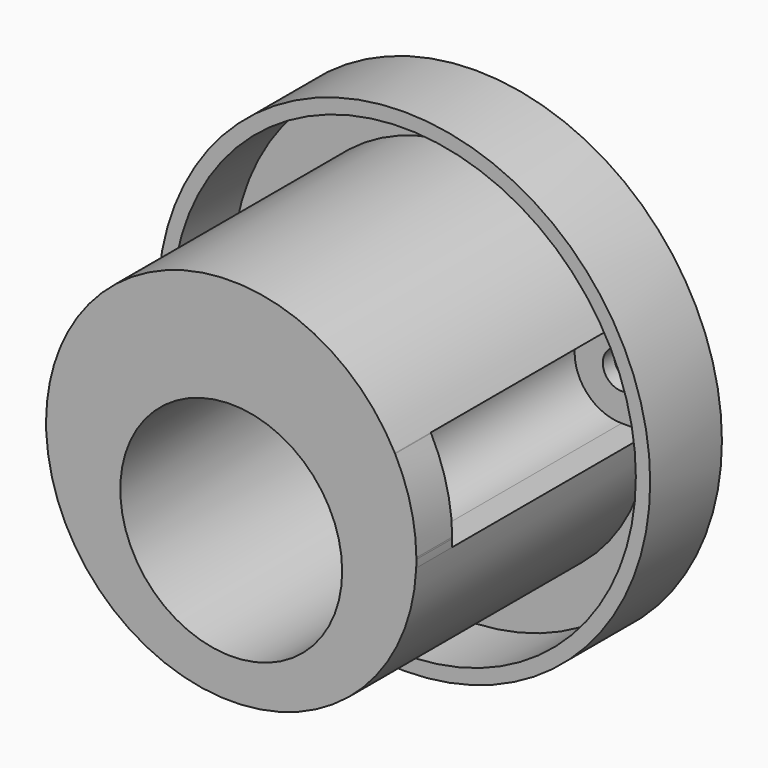
from build123d import *

# Parameters (mm, degrees)
F0_R     = 25.85
F0_R_2   = 4.9
F0_R_3   = 2.1
F1_DEPTH = 1.6
F0_R_4   = 27.45
F2_DEPTH = 10
F3_R     = 12.375
F4_DEPTH = 32.5
F6_DEPTH = 5


# Not quite as in the source:
# - ends of sketch curves that miss each other by under 0.0002 mm in the source are joined


with BuildPart() as f1:
    # F0 (on Front) → F1 (new body)
    with BuildSketch(Plane.XZ):
        Circle(F0_R)
        with Locations((0, -3.85)):
            Circle(F0_R_2, mode=Mode.SUBTRACT)
        with Locations((-17.55, 4.4)):
            Circle(F0_R_3, mode=Mode.SUBTRACT)
        with Locations((17.55, 4.4)):
            Circle(F0_R_3, mode=Mode.SUBTRACT)
    extrude(amount=F1_DEPTH)

    # F0 (on Front) → F2 (join)
    with BuildSketch(Plane.XZ):
        Circle(F0_R_4)
        Circle(F0_R, mode=Mode.SUBTRACT)
    extrude(amount=F2_DEPTH)

    # F3 (on face) → F4 (join)
    with BuildSketch(Plane.XZ.offset(1.6)):
        with BuildLine():
            Line((17.55, 9.65), (18.2565056898, 9.65))
            ThreePointArc((18.2565056898, 9.65), (0, 20.65), (-18.2565056898, 9.65))
            Line((-18.2565056898, 9.65), (-17.55, 9.65))
            ThreePointArc((-17.55, 9.65), (-13.8376893988, 8.1123106012), (-12.3, 4.4))
            ThreePointArc((-12.3, 4.4), (-13.8376893988, 0.6876893988), (-17.55, -0.85))
            Line((-17.55, -0.85), (-20.6324986369, -0.85))
            ThreePointArc((-20.6324986369, -0.85), (0, -20.65), (20.6324986369, -0.85))
            Line((20.6324986369, -0.85), (17.55, -0.85))
            ThreePointArc((17.55, -0.85), (12.3, 4.4), (17.55, 9.65))
        make_face()
        with Locations((0, -3.85)):
            Circle(F3_R, mode=Mode.SUBTRACT)
    extrude(amount=F4_DEPTH)

    # F5 (on face) → F6 (join)
    with BuildSketch(Plane.XZ.offset(34.1)):
        with BuildLine():
            ThreePointArc((-17.55, -0.85), (-13.8376893988, 0.6876893988), (-12.3, 4.4))
            ThreePointArc((-12.3, 4.4), (-13.8376893988, 8.1123106012), (-17.55, 9.65))
            ThreePointArc((-17.55, 9.65), (-17.9177743439, 9.6371024462), (-18.2837416824, 9.598473155))
            ThreePointArc((-18.2837416824, 9.598473155), (-20.0300885135, 5.0217580727), (-20.6493606667, 0.1624932498))
            ThreePointArc((-20.6493606667, 0.1624932498), (-19.1802744495, -0.5904614235), (-17.55, -0.85))
        make_face()
        with BuildLine():
            ThreePointArc((-18.2837416824, 9.598473155), (-17.9177743439, 9.6371024462), (-17.55, 9.65))
            Line((-17.55, 9.65), (-18.2565056898, 9.65))
            ThreePointArc((-18.2565056898, 9.65), (-18.2701054669, 9.6242270457), (-18.2837416824, 9.598473155))
        make_face()
        with BuildLine():
            Line((-20.6324986369, -0.85), (-17.55, -0.85))
            ThreePointArc((-17.55, -0.85), (-19.1802744495, -0.5904614235), (-20.6493606667, 0.1624932498))
            ThreePointArc((-20.6493606667, 0.1624932498), (-20.6471369089, -0.3438567505), (-20.6324986369, -0.85))
        make_face()
        with BuildLine():
            ThreePointArc((20.6493606667, 0.1624932498), (20.0300885135, 5.0217580727), (18.2836688601, 9.5984349253))
            ThreePointArc((18.2836688601, 9.5984349253), (17.9177743439, 9.6371024462), (17.55, 9.65))
            ThreePointArc((17.55, 9.65), (12.3, 4.4), (17.55, -0.85))
            ThreePointArc((17.55, -0.85), (19.1802744495, -0.5904614235), (20.6493606667, 0.1624932498))
        make_face()
        with BuildLine():
            Line((17.55, -0.85), (20.6324986369, -0.85))
            ThreePointArc((20.6324986369, -0.85), (20.6456241956, -0.425090078), (20.65, 0))
            ThreePointArc((20.65, 0), (20.6498401661, 0.0812472538), (20.6493606667, 0.1624932498))
            ThreePointArc((20.6493606667, 0.1624932498), (19.1802744495, -0.5904614235), (17.55, -0.85))
        make_face()
        with BuildLine():
            ThreePointArc((18.2836688601, 9.5984349253), (18.2701054669, 9.6242270457), (18.2565056898, 9.65))
            Line((18.2565056898, 9.65), (17.55, 9.65))
            ThreePointArc((17.55, 9.65), (17.9177743439, 9.6371024462), (18.2836688601, 9.5984349253))
        make_face()
    extrude(amount=-F6_DEPTH)


solid = f1.part
